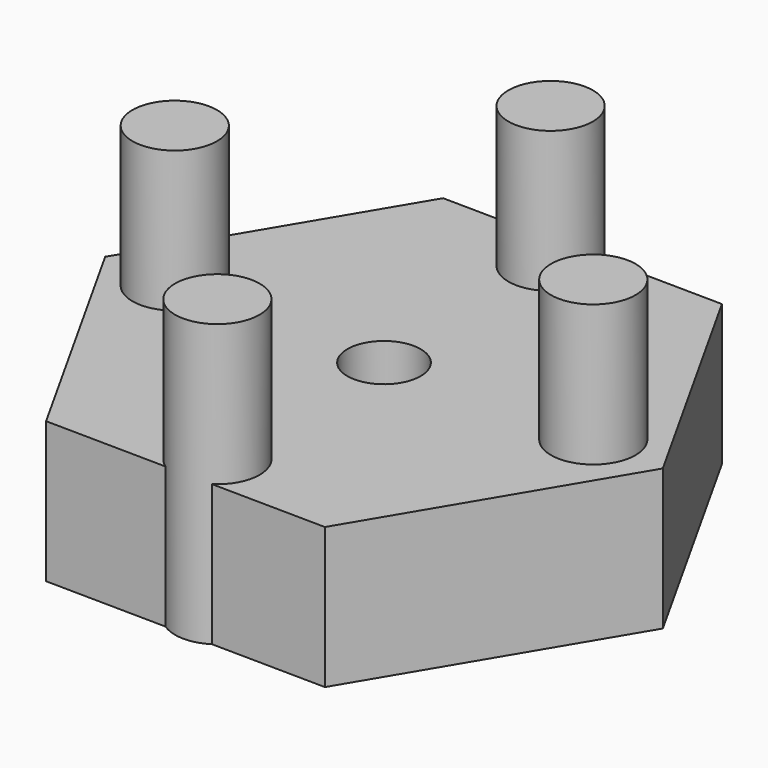
from build123d import *

# Parameters (mm, degrees)
F0_R     = 3.81
F1_DEPTH = 12.7
F2_R     = 3.302
F3_DEPTH = 25.4
F4_DEPTH = 25.4


# Not quite as in the source:
# - a feature names something its author has since deleted; it is built from what else it names


with BuildPart() as f1:
    # F0 (on Top) → F1 (new body)
    with BuildSketch(Plane.XY):
        with BuildLine():
            Line((2.1058679478, -22.0272163702), (12.4043320804, -22.1651200231))
            Line((12.4043320804, -22.1651200231), (25.3977230582, -0.3400933129))
            Line((25.3977230582, -0.3400933129), (12.9933909777, 21.8250267102))
            Line((12.9933909777, 21.8250267102), (2.1058679478, 21.9708182746))
            ThreePointArc((2.1058679478, 21.9708182746), (3.3265702822, 20.6034553453), (3.7674883359, 18.8243019401))
            ThreePointArc((3.7674883359, 18.8243019401), (-1.8666159044, 15.4793439852), (-2.1058679478, 22.0272163702))
            Line((-2.1058679478, 22.0272163702), (-12.4043320804, 22.1651200231))
            Line((-12.4043320804, 22.1651200231), (-25.3977230582, 0.3400933129))
            Line((-25.3977230582, 0.3400933129), (-12.9933909777, -21.8250267102))
            Line((-12.9933909777, -21.8250267102), (-2.1058679478, -21.9708182746))
            ThreePointArc((-2.1058679478, -21.9708182746), (-1.7366417411, -15.4552199938), (3.8525116641, -18.8243019401))
            ThreePointArc((3.8525116641, -18.8243019401), (3.3874696191, -20.6484061804), (2.1058679478, -22.0272163702))
        make_face()
        with Locations((-18.8243019401, -0.0425116641)):
            Circle(F0_R, mode=Mode.SUBTRACT)
        with Locations((18.8243019401, 0.0425116641)):
            Circle(F0_R, mode=Mode.SUBTRACT)
        with BuildLine():
            ThreePointArc((-2.1058679478, -21.9708182746), (-0.0085023328, -22.6339603988), (2.1058679478, -22.0272163702))
            Line((2.1058679478, -22.0272163702), (-2.1058679478, -21.9708182746))
        make_face()
        with BuildLine():
            Line((-2.1058679478, -21.9708182746), (2.1058679478, -22.0272163702))
            ThreePointArc((2.1058679478, -22.0272163702), (3.3874696191, -20.6484061804), (3.8525116641, -18.8243019401))
            ThreePointArc((3.8525116641, -18.8243019401), (-1.7366417411, -15.4552199938), (-2.1058679478, -21.9708182746))
        make_face()
        with BuildLine():
            ThreePointArc((3.7674883359, 18.8243019401), (3.3265702822, 20.6034553453), (2.1058679478, 21.9708182746))
            Line((2.1058679478, 21.9708182746), (-2.1058679478, 22.0272163702))
            ThreePointArc((-2.1058679478, 22.0272163702), (-1.8666159044, 15.4793439852), (3.7674883359, 18.8243019401))
        make_face()
        with BuildLine():
            Line((-2.1058679478, 22.0272163702), (2.1058679478, 21.9708182746))
            ThreePointArc((2.1058679478, 21.9708182746), (0.0085023328, 22.6339603988), (-2.1058679478, 22.0272163702))
        make_face()
    extrude(amount=F1_DEPTH)

    # F2 (on face) → F3 (cut)
    with BuildSketch(Plane.XY.offset(12.7)):
        Circle(F2_R)
    extrude(amount=-F3_DEPTH, mode=Mode.SUBTRACT)

    # F0 (on Top) → F4 (join)
    with BuildSketch(Plane.XY):
        with BuildLine():
            Line((-2.1058679478, 22.0272163702), (2.1058679478, 21.9708182746))
            ThreePointArc((2.1058679478, 21.9708182746), (0.0085023328, 22.6339603988), (-2.1058679478, 22.0272163702))
        make_face()
        with BuildLine():
            ThreePointArc((3.7674883359, 18.8243019401), (3.3265702822, 20.6034553453), (2.1058679478, 21.9708182746))
            Line((2.1058679478, 21.9708182746), (-2.1058679478, 22.0272163702))
            ThreePointArc((-2.1058679478, 22.0272163702), (-1.8666159044, 15.4793439852), (3.7674883359, 18.8243019401))
        make_face()
        with Locations((18.8243019401, 0.0425116641)):
            Circle(F0_R)
        with BuildLine():
            ThreePointArc((-2.1058679478, -21.9708182746), (-0.0085023328, -22.6339603988), (2.1058679478, -22.0272163702))
            Line((2.1058679478, -22.0272163702), (-2.1058679478, -21.9708182746))
        make_face()
        with BuildLine():
            Line((-2.1058679478, -21.9708182746), (2.1058679478, -22.0272163702))
            ThreePointArc((2.1058679478, -22.0272163702), (3.3874696191, -20.6484061804), (3.8525116641, -18.8243019401))
            ThreePointArc((3.8525116641, -18.8243019401), (-1.7366417411, -15.4552199938), (-2.1058679478, -21.9708182746))
        make_face()
        with Locations((-18.8243019401, -0.0425116641)):
            Circle(F0_R)
    extrude(amount=F4_DEPTH)


solid = f1.part
